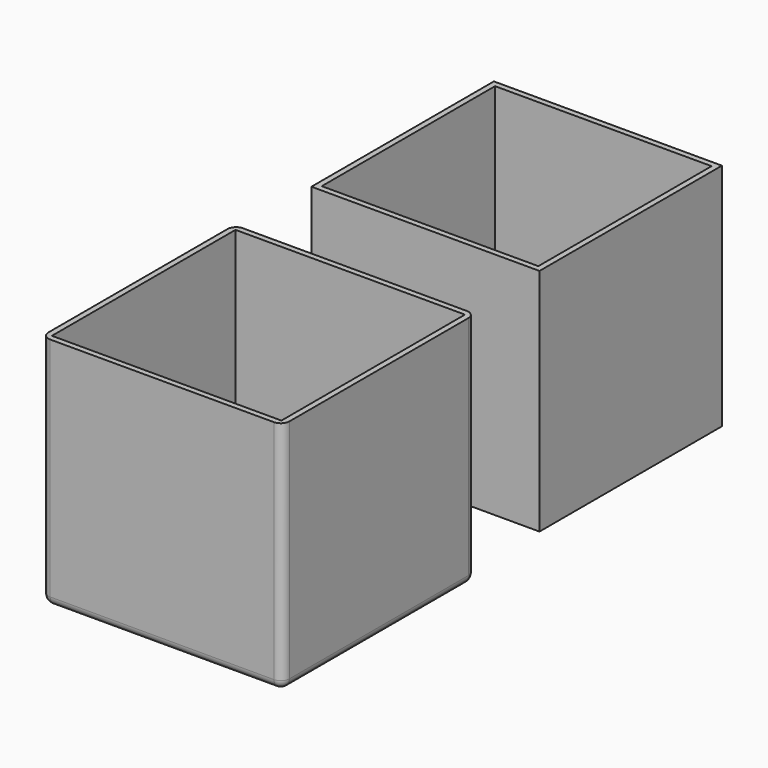
from build123d import *

# Parameters (mm, degrees)
F0_W         = 80
F0_H         = 80
F1_DEPTH     = 80
F2_T         = 2
F3_W         = 79.5
F3_H         = 79.5
F4_DEPTH     = 80
F5_T         = -2
F6_T1_DEPTH  = 86.5
F6_T3_DEPTH  = 78
F6_T5_DEPTH  = 78
F6_S9_W      = 3
F6_S9_H      = 3
F6_T10_DEPTH = 3
F6_S15_W     = 3
F6_S15_H     = 3
F6_T16_DEPTH = 3
F6_S21_W     = 3
F6_S21_H     = 3
F6_T22_DEPTH = 3
F6_S27_W     = 3
F6_S27_H     = 3
F6_T28_DEPTH = 3
F8_R         = 2.5
F9_DEPTH     = 2.05


# Not quite as in the source:
# - a fillet or chamfer that OpenCascade refuses, or shapes differently, is made with other operations: its cross-section is extruded or revolved along the edge and cut away or added
# - a feature of the source that left no trace in its solid (it failed there, or was rolled back) is left out


with BuildPart() as f1:
    # F0 (on Top) → F1 (new body)
    with BuildSketch(Plane.XY):
        Rectangle(F0_W, F0_H)
    extrude(amount=F1_DEPTH)

    # F2
    f2_openings = [f1.faces().sort_by_distance(p)[0] for p in [
        (0, 0, 80),
    ]]
    offset(amount=F2_T, openings=f2_openings, kind=Kind.INTERSECTION)

    # F6: fillet of radius 3 on 8 edges, made by hand

    # F6_s2 → F6_t1 (cut)
    with BuildSketch(Plane.XY.offset(1)):
        with BuildLine():
            ThreePointArc((42, -39), (41.1213203436, -41.1213203436), (39, -42))
            Line((39, -42), (42, -42))
            Line((42, -42), (42, -39))
        make_face()
        with BuildLine():
            ThreePointArc((42, 39), (41.1213203436, 41.1213203436), (39, 42))
            Line((39, 42), (42, 42))
            Line((42, 42), (42, 39))
        make_face()
        with BuildLine():
            ThreePointArc((-39, 42), (-41.1213203436, 41.1213203436), (-42, 39))
            Line((-42, 39), (-42, 42))
            Line((-42, 42), (-39, 42))
        make_face()
        with BuildLine():
            ThreePointArc((-42, -39), (-41.1213203436, -41.1213203436), (-39, -42))
            Line((-39, -42), (-42, -42))
            Line((-42, -42), (-42, -39))
        make_face()
    extrude(amount=F6_T1_DEPTH, mode=Mode.SUBTRACT)

    # F6_s4 → F6_t3 (cut)
    with BuildSketch(Plane.XZ.offset(-39)):
        with BuildLine():
            ThreePointArc((42, 1), (41.1213203436, -1.1213203436), (39, -2))
            Line((39, -2), (42, -2))
            Line((42, -2), (42, 1))
        make_face()
        with BuildLine():
            ThreePointArc((-42, 1), (-41.1213203436, -1.1213203436), (-39, -2))
            Line((-39, -2), (-42, -2))
            Line((-42, -2), (-42, 1))
        make_face()
    extrude(amount=F6_T3_DEPTH, mode=Mode.SUBTRACT)

    # F6_s6 → F6_t5 (cut)
    with BuildSketch(Plane.YZ.offset(-39)):
        with BuildLine():
            ThreePointArc((42, 1), (41.1213203436, -1.1213203436), (39, -2))
            Line((39, -2), (42, -2))
            Line((42, -2), (42, 1))
        make_face()
        with BuildLine():
            ThreePointArc((-42, 1), (-41.1213203436, -1.1213203436), (-39, -2))
            Line((-39, -2), (-42, -2))
            Line((-42, -2), (-42, 1))
        make_face()
    extrude(amount=F6_T5_DEPTH, mode=Mode.SUBTRACT)


with BuildPart() as f4:
    # F3 (on Top) → F4 (new body)
    with BuildSketch(Plane.XY):
        with Locations((0, 112.5286910326)):
            Rectangle(F3_W, F3_H)
    extrude(amount=F4_DEPTH)

    # F5
    f5_openings = [f4.faces().sort_by_distance(p)[0] for p in [
        (0, 112.528691, 80),
    ]]
    offset(amount=F5_T, openings=f5_openings)

    # F8 (on face) → F9 (cut)
    with BuildSketch(Plane(origin=(0, 0, 0), x_dir=(1, 0, 0), z_dir=(0, 0, -1))):
        with Locations((20.5125, -133.0411910326)):
            Circle(F8_R)
        with Locations((-20.5125, -133.0411910326)):
            Circle(F8_R)
        with Locations((-20.5125, -92.0161910326)):
            Circle(F8_R)
        with Locations((0, -112.5286910326)):
            Circle(F8_R)
        with Locations((20.5125, -92.0161910326)):
            Circle(F8_R)
    extrude(amount=-F9_DEPTH, mode=Mode.SUBTRACT)


with BuildPart() as f6_tool8:
    # F6_s9 → F6_t10 (new body)
    with BuildSketch(Plane.XZ.offset(39)):
        with Locations((40.5, -0.5)):
            Rectangle(F6_S9_W, F6_S9_H)
    extrude(amount=F6_T10_DEPTH)

    # F6_s11 → F6_t12 (revolve, cut)
    with BuildSketch(Plane(origin=(39, -39, 1), x_dir=(-0.7071067812, 0, 0.7071067812), z_dir=(0.7071067812, 0, 0.7071067812))):
        with BuildLine():
            ThreePointArc((0, -3), (3, 0), (0, 3))
            Line((0, 3), (0, -3))
        make_face()
    revolve(axis=Axis((39, -39, 1), (0, -1, 0)), mode=Mode.SUBTRACT)


with BuildPart() as f1_1:
    add(f1.part)

    # F6_t7: cut F6_tool8
    add(f6_tool8.part, mode=Mode.SUBTRACT)


with BuildPart() as f6_tool14:
    # F6_s15 → F6_t16 (new body)
    with BuildSketch(Plane.XY.offset(1)):
        with Locations((40.5, 40.5)):
            Rectangle(F6_S15_W, F6_S15_H)
    extrude(amount=-F6_T16_DEPTH)

    # F6_s17 → F6_t18 (revolve, cut)
    with BuildSketch(Plane(origin=(39, 39, 1), x_dir=(-0.7071067812, -0.7071067812, 0), z_dir=(0.7071067812, -0.7071067812, 0))):
        with BuildLine():
            ThreePointArc((0, -3), (3, 0), (0, 3))
            Line((0, 3), (0, -3))
        make_face()
    revolve(axis=Axis((39, 39, 1), (0, 0, -1)), mode=Mode.SUBTRACT)


with BuildPart() as f1_2:
    add(f1_1.part)

    # F6_t13: cut F6_tool14
    add(f6_tool14.part, mode=Mode.SUBTRACT)


with BuildPart() as f6_tool20:
    # F6_s21 → F6_t22 (new body)
    with BuildSketch(Plane.YZ.offset(-39)):
        with Locations((40.5, -0.5)):
            Rectangle(F6_S21_W, F6_S21_H)
    extrude(amount=-F6_T22_DEPTH)

    # F6_s23 → F6_t24 (revolve, cut)
    with BuildSketch(Plane(origin=(-39, 39, 1), x_dir=(0, -0.7071067812, 0.7071067812), z_dir=(0, -0.7071067812, -0.7071067812))):
        with BuildLine():
            ThreePointArc((0, -3), (3, 0), (0, 3))
            Line((0, 3), (0, -3))
        make_face()
    revolve(axis=Axis((-39, 39, 1), (-1, 0, 0)), mode=Mode.SUBTRACT)


with BuildPart() as f1_3:
    add(f1_2.part)

    # F6_t19: cut F6_tool20
    add(f6_tool20.part, mode=Mode.SUBTRACT)


with BuildPart() as f6_tool26:
    # F6_s27 → F6_t28 (new body)
    with BuildSketch(Plane.YZ.offset(-39)):
        with Locations((-40.5, -0.5)):
            Rectangle(F6_S27_W, F6_S27_H)
    extrude(amount=-F6_T28_DEPTH)

    # F6_s29 → F6_t30 (revolve, cut)
    with BuildSketch(Plane(origin=(-39, -39, 1), x_dir=(0, 0.7071067812, 0.7071067812), z_dir=(0, -0.7071067812, 0.7071067812))):
        with BuildLine():
            ThreePointArc((0, -3), (3, 0), (0, 3))
            Line((0, 3), (0, -3))
        make_face()
    revolve(axis=Axis((-39, -39, 1), (-1, 0, 0)), mode=Mode.SUBTRACT)


with BuildPart() as f1_4:
    add(f1_3.part)

    # F6_t25: cut F6_tool26
    add(f6_tool26.part, mode=Mode.SUBTRACT)


solid = Compound([f4.part, f1_4.part])
